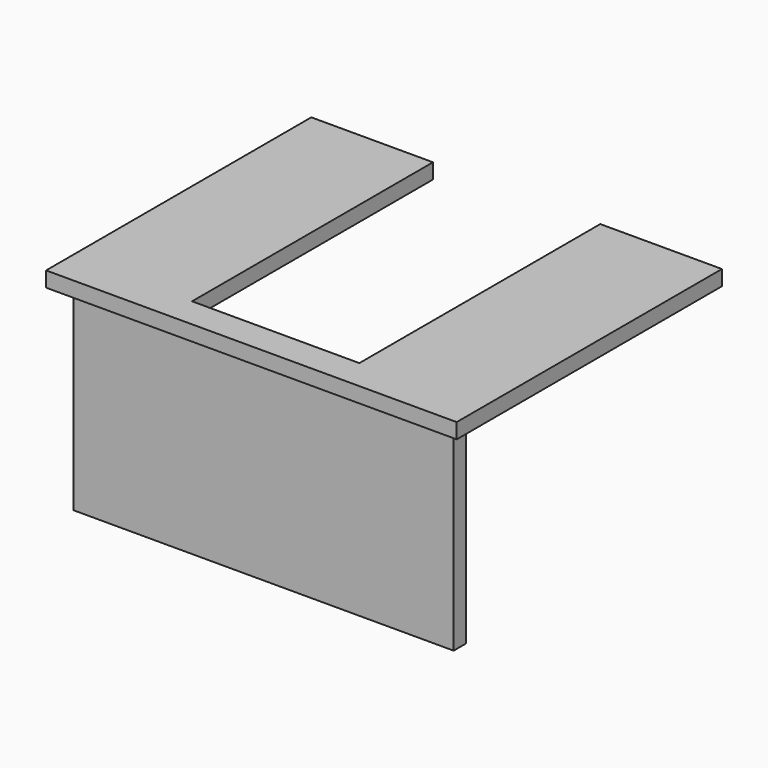
from build123d import *

# Parameters (mm, degrees)
F0_W      = 50.8
F0_H      = 50.8
F1_DEPTH  = 1005.84
F3_DEPTH  = 50.8
F4_W      = 1371.6
F4_H      = 50.8
F5_DEPTH  = 50.8
F11_DEPTH = 955.04


# Not quite as in the source:
# - a feature of the source that left no trace in its solid (it failed there, or was rolled back) is left out


with BuildPart() as f1:
    # F0 (on Front) → F1 (new body)
    with BuildSketch(Plane.XZ):
        with Locations((-1295.4, 683.9833942235)):
            Rectangle(F0_W, F0_H)
        with Locations((25.4, 683.9833942235)):
            Rectangle(F0_W, F0_H)
        Polygon((-1270, 0), (0, 0), (0, 658.5833942235), (0, 709.3833942235), (-1270, 709.3833942235), (-1270, 658.5833942235), align=None)
    extrude(amount=-F1_DEPTH)

    # F2 (on face) → F3 (join)
    with BuildSketch(Plane(origin=(0, 1005.84, 0), x_dir=(-1, 0, 0), z_dir=(0, 1, 0))):
        Polygon((1320.8, 709.3833942235), (914.4, 709.3833942235), (914.4, 658.5833942235), (1270, 658.5833942235), (1320.8, 658.5833942235), align=None)
        Polygon((-50.8, 709.3833942235), (-50.8, 658.5833942235), (0, 658.5833942235), (355.6, 658.5833942235), (355.6, 709.3833942235), align=None)
    extrude(amount=F3_DEPTH)

    # F4 (on face) → F5 (join)
    with BuildSketch(Plane.XZ):
        with Locations((-635, 683.9833942235)):
            Rectangle(F4_W, F4_H)
    extrude(amount=F5_DEPTH)

    # F10 (on face) → F11 (cut)
    with BuildSketch(Plane(origin=(0, 1005.84, 0), x_dir=(-1, 0, 0), z_dir=(0, 1, 0))):
        Polygon((355.6, 709.3833942235), (355.6, 658.5833942235), (355.6, 113.7688308954), (914.4, 113.7688308954), (914.4, 658.5833942235), (914.4, 709.3833942235), align=None)
        Polygon((355.6, 113.7688308954), (355.6, 658.5833942235), (0, 658.5833942235), (0, 0), (1270, 0), (1270, 658.5833942235), (914.4, 658.5833942235), (914.4, 113.7688308954), align=None)
    extrude(amount=-F11_DEPTH, mode=Mode.SUBTRACT)


solid = f1.part
